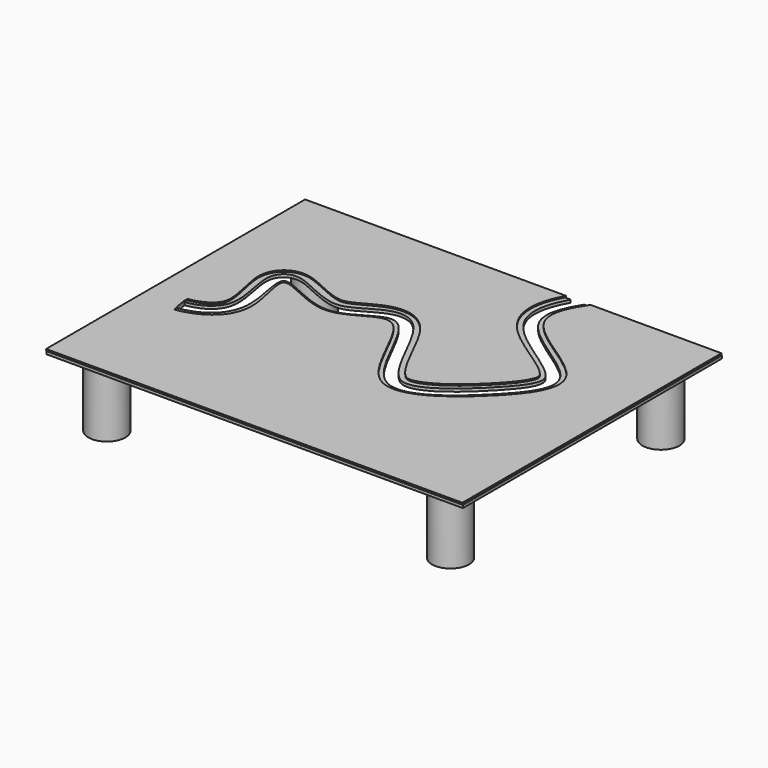
from build123d import *

# Parameters (mm, degrees)
F0_W          = 900
F0_H          = 700
F2_DEPTH      = 3
F3_DEPTH      = 25
F3_DEPTH_BACK = 25
F6_DEPTH      = 25
F6_DEPTH_BACK = 25
F7_W          = 900
F7_H          = 700
F9_DEPTH      = 6
F11_R         = 40
F12_DEPTH     = 150


# Not quite as in the source:
# - the dataset's text gives a spline's control points without its knots; the knots are read off the source's solid


with BuildPart() as f2:
    # F0 (on Top) → F2 (new body)
    with BuildSketch(Plane.XY):
        with Locations((136.779838565, 140.37967287)):
            Rectangle(F0_W, F0_H)
    extrude(amount=F2_DEPTH)

    # F1 (on Top) → F3 (cut, two sides)
    with BuildSketch(Plane.XY) as f3_sk:
        with BuildLine():
            Line((-241.4856788522, 82.2124957097), (-234.3062907457, 37.7888940275))
            add(Edge.make_bspline(
                [(-234.3062907457, 37.7888940275), (-183.2200698821, 46.0450414938), (-107.8197896412, 102.2279372719), (-192.2750551174, 283.579620296), (-24.0171318012, 149.9224145171), (99.4434854713, 307.8000943084), (175.8744786158, -38.137750164), (392.3120352571, 121.8215640239), (495.7588052716, 272.9639793915), (212.09229922, 380.1642280608), (301.8253737576, 491.1332534511), (345.4286754131, 545.0569987297)],
                knots=[0, 0, 0, 0, 0.1005186811, 0.1948714664, 0.2944457767, 0.3919205483, 0.524446972, 0.6500546131, 0.7560619639, 0.8852543369, 1, 1, 1, 1], degree=3))
            Line((345.4286754131, 545.0569987297), (310.4370311075, 573.3516064985))
            add(Edge.make_bspline(
                [(-241.4856788522, 82.2124957097), (-235.5376995244, 83.1737606775), (-227.1834080935, 85.1443072797), (-217.474364878, 88.6042185531), (-210.9663273096, 91.5416769635), (-205.2747075425, 94.7414795634), (-200.4160544418, 98.1187472011), (-196.373293023, 101.5953254918), (-193.0908775239, 105.1164927775), (-190.4790946185, 108.673215132), (-188.772395717, 111.7142206402), (-187.6443639611, 114.2600259837), (-186.91078749, 116.2492961693), (-186.2869465038, 118.3436017222), (-185.8604232074, 120.1988345417), (-185.5789375302, 121.7627021332), (-185.3991590865, 122.9783217928), (-185.252302169, 124.2414938638), (-185.1405994233, 125.5490498855), (-185.059563113, 126.9970714119), (-185.0000994287, 129.0879426638), (-185.0248632154, 131.9899533939), (-185.2286698235, 135.8675595467), (-185.6086882806, 140.0794825573), (-186.1581698074, 144.5682595729), (-187.0987121971, 150.8533570489), (-188.6205679067, 159.1522141918), (-190.8240279465, 169.5043124094), (-192.8083784067, 178.2695336381), (-194.3818406654, 185.3095616522), (-195.5285456157, 190.6070149505), (-196.6143456264, 195.9387036323), (-197.6084875244, 201.3452092887), (-198.4727294543, 206.9018156809), (-199.1496740668, 212.7389962035), (-199.4764712019, 218.0162233827), (-199.4894720296, 222.6632212336), (-199.3258979633, 226.4234804566), (-198.919614654, 230.5290516319), (-198.1659289654, 235.0572516522), (-196.9118918995, 240.0783575162), (-194.9451306123, 245.6253274688), (-192.4879995558, 250.6392221678), (-189.898614037, 254.7703034363), (-187.6218228143, 257.8777610524), (-184.9992992364, 260.934338153), (-182.0377655849, 263.8704376875), (-179.3129029064, 266.1548327791), (-177.000331504, 267.8542399638), (-174.6237907367, 269.4492377395), (-171.6062006951, 271.2068826251), (-167.9761634622, 272.9460428746), (-164.409661789, 274.3311498765), (-159.8065692755, 275.749902793), (-154.4349269126, 276.8203829827), (-148.7149350442, 277.3109893938), (-143.6791934777, 277.2781780434), (-139.2282351443, 276.9098327801), (-135.2505889333, 276.3274056454), (-131.6452560188, 275.6060761092), (-128.327829438, 274.7915830848), (-124.1994201874, 273.6177648935), (-119.454378243, 272.0297965106), (-114.1330202601, 269.9985841874), (-109.0163936944, 267.8708559657), (-104.0042481448, 265.6683344255), (-99.0398525291, 263.4119036969), (-94.0934068391, 261.1245526128), (-87.5071738324, 258.0675515109), (-79.2894636179, 254.301217329), (-69.5603592504, 250.1084557216), (-61.7384184503, 247.0939974118), (-55.7995425295, 245.0842808334), (-51.5499774528, 243.8013204219), (-47.5536122712, 242.7614646682), (-43.8633351999, 241.9756441117), (-41.0890345702, 241.5330763696), (-39.0767461943, 241.2996839349), (-37.6771518248, 241.1816399507), (-36.3922517161, 241.116479596), (-35.4214542607, 241.1018193712), (-34.7043651988, 241.1108325263), (-34.2011207672, 241.1268350515), (-33.6853437819, 241.1532206705), (-32.9848262391, 241.2026104861), (-32.080215541, 241.2918119898), (-30.9425191435, 241.4457711216), (-29.747492374, 241.6498724502), (-28.0732155104, 241.9930222828), (-25.822720168, 242.5627626208), (-21.880330047, 243.7981397699), (-16.331982542, 245.9761062402), (-8.8118359212, 249.5607949136), (-0.5434559099, 253.9526763782), (8.4508129905, 258.9262639267), (16.6403545663, 263.3417972682), (23.7599841554, 266.8841366803), (29.4467345634, 269.4962211057), (35.5566372376, 272.0010306462), (42.1823374373, 274.311405811), (49.4236395705, 276.3023826176), (57.3672041666, 277.795696083), (66.0465099256, 278.5509411968), (75.3837631228, 278.2821676865), (83.5113265637, 276.9778692101), (89.2081655274, 275.4330144664), (92.4367063904, 274.3708027239), (94.8382851466, 273.4852798104), (96.8161375588, 272.6754654295), (98.3841938016, 271.9843530185), (99.9262943401, 271.2721286966), (101.8038878917, 270.3453559302), (104.702705147, 268.7934917732), (108.1317869173, 266.7405344791), (111.9541425106, 264.1395026786), (115.5087239258, 261.4346763787), (119.927069824, 257.7228957042), (124.9169432693, 252.9328275462), (130.2508034542, 247.026543135), (135.0896327978, 240.9927455699), (139.554556696, 234.8416200953), (145.1283850319, 226.4875741975), (151.5589218926, 215.7632245239), (158.7710272688, 202.497891756), (165.6801971146, 188.9538806141), (172.4151365402, 175.2994869993), (179.0582911899, 161.7422451206), (185.660525585, 148.5206349377), (192.2444338178, 135.8994918833), (198.8008182512, 124.1678836236), (205.2768380346, 113.6369815809), (210.5101981, 106.1358052224), (214.4899104198, 101.0609993718), (217.3303617383, 97.7534217065), (219.978464374, 94.9733838681), (222.3765020584, 92.7378899598), (224.1137016073, 91.3274700325), (225.3142899389, 90.4567825785), (226.1163341361, 89.924057213), (226.8029845386, 89.5091405515), (227.4733439715, 89.1430138534), (228.1291176651, 88.822150909), (228.9996846256, 88.4432304879), (230.1054945245, 88.0467609434), (231.54537094, 87.6664964427), (233.1753732843, 87.3794091452), (235.057273097, 87.2021281247), (237.2335796296, 87.1635396823), (240.55731177, 87.3413929062), (245.5227987888, 88.079008451), (252.6791739242, 89.9923664451), (260.8301872351, 93.0264381942), (269.7570797741, 97.1825815618), (279.2556215065, 102.4009159936), (289.1468102787, 108.584934908), (299.2760739512, 115.6176345184), (309.5093899796, 123.3712014191), (319.7287874812, 131.7124258746), (329.8286859902, 140.5058445218), (338.0648038503, 148.0964177817), (344.5013770548, 154.2589683131), (348.4500767297, 158.1321041895), (351.5636214838, 161.2392515861), (354.6286384304, 164.3330415235), (358.3546871655, 168.163507658), (362.6480774345, 172.6981225537), (368.1173165148, 178.6510472941), (374.4439024175, 185.8985119346), (381.1201011492, 194.2088317575), (386.7882817119, 202.0338405705), (391.3723846707, 209.2487053252), (394.8283570488, 215.7004013288), (397.1689795838, 221.2164346332), (398.274140703, 224.8961691748), (398.7586304729, 227.2523477751), (398.9589780282, 228.7346603805), (399.033607176, 229.9543070221), (399.0177225056, 230.952451348), (398.9374713249, 231.7885688151), (398.8035372952, 232.5375385066), (398.6059933192, 233.282855915), (398.3615456687, 233.9702274749), (398.0917291127, 234.596295897), (397.885446547, 235.0253148368), (397.6933380765, 235.3947640399), (397.5351601954, 235.6845823574), (397.3594254936, 235.9919532357), (397.0874783947, 236.4470374628), (396.679784191, 237.0891477727), (395.8733663132, 238.2656919148), (394.567493912, 239.9926785021), (392.5131211223, 242.4074256407), (389.137265676, 246.0021498199), (383.7741089396, 251.0640022626), (375.751488869, 257.7405013236), (366.417496646, 264.8362812315), (356.0404038889, 272.2467658517), (344.8731898776, 279.9209527707), (333.1509121216, 287.8448474083), (321.0910339513, 296.0335168672), (308.893794176, 304.5289467569), (296.7425913103, 313.4033633299), (284.8049272706, 322.7684284522), (273.237915057, 332.7926592747), (264.0409228143, 341.9040126463), (257.0563649981, 349.8326975335), (252.0449681123, 356.1585682546), (248.1020472958, 361.7995109897), (245.1253394442, 366.5665889108), (242.9935925432, 370.2770521418), (241.3129881952, 373.4859400827), (240.0325980452, 376.1290050305), (238.8113517142, 378.7924683854), (237.3946194858, 382.1615894078), (235.3686208631, 387.6220814248), (233.2949562773, 394.552809555), (231.546773022, 402.9453959487), (230.5193972595, 411.3225036077), (230.1719914596, 419.6044271535), (230.4480888242, 427.7291455333), (231.5621988176, 438.2982923287), (234.1862414869, 450.9526422368), (238.8303853448, 465.2427656184), (244.6130062197, 478.7677873011), (251.2809191489, 491.6831883403), (258.6500420567, 504.1296805595), (266.5761934981, 516.2184522105), (274.935846315, 528.0312592745), (283.6149215817, 539.6249662726), (295.464949001, 554.8390039644), (304.4995700078, 566.0088107058), (310.4370311075, 573.3516064985)],
                knots=[0, 0, 0, 0, 0.015625, 0.0234375, 0.03125, 0.0390625, 0.046875, 0.0546875, 0.0625, 0.0703125, 0.078125, 0.08203125, 0.0859375, 0.08984375, 0.09375, 0.095703125, 0.09765625, 0.099609375, 0.1015625, 0.103515625, 0.10546875, 0.109375, 0.11328125, 0.1171875, 0.12109375, 0.125, 0.1328125, 0.140625, 0.1484375, 0.15234375, 0.15625, 0.16015625, 0.1640625, 0.16796875, 0.171875, 0.17578125, 0.177734375, 0.1796875, 0.181640625, 0.18359375, 0.185546875, 0.1875, 0.189453125, 0.1904296875, 0.19140625, 0.1923828125, 0.193359375, 0.1943359375, 0.1948242188, 0.1953125, 0.1962890625, 0.197265625, 0.1982421875, 0.19921875, 0.201171875, 0.203125, 0.205078125, 0.20703125, 0.208984375, 0.2109375, 0.212890625, 0.21484375, 0.21875, 0.22265625, 0.2265625, 0.23046875, 0.234375, 0.23828125, 0.2421875, 0.25, 0.2578125, 0.265625, 0.26953125, 0.2734375, 0.27734375, 0.28125, 0.28515625, 0.287109375, 0.2890625, 0.291015625, 0.29296875, 0.2939453125, 0.294921875, 0.2958984375, 0.296875, 0.298828125, 0.30078125, 0.302734375, 0.3046875, 0.30859375, 0.3125, 0.3203125, 0.328125, 0.3359375, 0.34375, 0.3515625, 0.35546875, 0.359375, 0.36328125, 0.3671875, 0.37109375, 0.375, 0.37890625, 0.3828125, 0.38671875, 0.388671875, 0.3896484375, 0.390625, 0.3916015625, 0.3920898438, 0.392578125, 0.3935546875, 0.39453125, 0.396484375, 0.3984375, 0.400390625, 0.40234375, 0.40625, 0.41015625, 0.4140625, 0.41796875, 0.421875, 0.4296875, 0.4375, 0.4453125, 0.453125, 0.4609375, 0.46875, 0.4765625, 0.484375, 0.4921875, 0.5, 0.50390625, 0.5078125, 0.51171875, 0.515625, 0.51953125, 0.521484375, 0.5234375, 0.525390625, 0.52734375, 0.529296875, 0.53125, 0.53515625, 0.5390625, 0.54296875, 0.546875, 0.55078125, 0.5546875, 0.5625, 0.5703125, 0.578125, 0.5859375, 0.59375, 0.6015625, 0.609375, 0.6171875, 0.625, 0.6328125, 0.640625, 0.64453125, 0.6484375, 0.650390625, 0.65234375, 0.65625, 0.66015625, 0.6640625, 0.671875, 0.6796875, 0.6875, 0.6953125, 0.703125, 0.7109375, 0.71875, 0.72265625, 0.7265625, 0.73046875, 0.734375, 0.73828125, 0.7421875, 0.74609375, 0.75, 0.751953125, 0.75390625, 0.7548828125, 0.755859375, 0.7568359375, 0.7578125, 0.759765625, 0.76171875, 0.765625, 0.76953125, 0.7734375, 0.78125, 0.7890625, 0.796875, 0.8046875, 0.8125, 0.8203125, 0.828125, 0.8359375, 0.84375, 0.8515625, 0.859375, 0.8671875, 0.87109375, 0.875, 0.87890625, 0.880859375, 0.8828125, 0.884765625, 0.8857421875, 0.88671875, 0.888671875, 0.890625, 0.89453125, 0.8984375, 0.90234375, 0.90625, 0.91015625, 0.9140625, 0.921875, 0.9296875, 0.9375, 0.9453125, 0.953125, 0.9609375, 0.96875, 0.9765625, 0.984375, 1, 1, 1, 1], degree=3))
        make_face()
    extrude(amount=F3_DEPTH, mode=Mode.SUBTRACT)
    extrude(f3_sk.sketch, amount=-F3_DEPTH_BACK, mode=Mode.SUBTRACT)


with BuildPart() as f2_1:
    # F5: moved
    add(f2.part.moved(Location((-139, -139, 6))))


with BuildPart() as f6:
    # F4 (on Top) → F6 (new body, two sides)
    with BuildSketch(Plane.XY) as f6_sk:
        with BuildLine():
            Line((-333.2689129169, -208.5999996712), (-329.2803639689, -233.2797783835))
            add(Edge.make_bspline(
                [(-329.2803639689, -233.2797783835), (-279.6440862088, -225.2579591544), (-215.0591975226, -169.0019007955), (-290.3221170229, 10.7279443108), (-115.933229477, -128.5278182105), (8.6171027688, 40.169951089), (91.4360122328, -317.6582258257), (294.4798541771, -146.0859910696), (390.4461045585, -16.0719332642), (105.2391975094, 95.5185231878), (204.8334747082, 217.5691570301), (250.45460219, 273.9883263187)],
                knots=[0, 0, 0, 0, 0.0976657324, 0.1914809372, 0.2938646504, 0.3927571199, 0.5271537272, 0.6507806642, 0.749994953, 0.8799442629, 1, 1, 1, 1], degree=3))
            Line((250.45460219, 273.9883263187), (231.014799798, 289.707552857))
            add(Edge.make_bspline(
                [(-333.2689129169, -208.5999996712), (-326.5356582324, -207.5118247648), (-317.1931037284, -205.2387950425), (-306.3838909726, -201.131018164), (-299.1159354338, -197.5685255044), (-292.6875905846, -193.5780513816), (-287.0795024379, -189.2040888935), (-282.2539728874, -184.4715031927), (-278.1616343726, -179.3755889151), (-274.7548284297, -173.8762725729), (-272.004457018, -167.9012394607), (-270.2621207217, -162.4489840488), (-269.3492323658, -158.3439603506), (-268.9196013639, -155.9107657182), (-268.6445813298, -154.0412952716), (-268.4179617417, -152.1250200421), (-268.2708607574, -150.4920692989), (-268.178315106, -149.1553098982), (-268.1017791313, -147.787649081), (-268.0366959253, -146.0273373624), (-268.0074636443, -143.83809812), (-268.0330013502, -140.8251744651), (-268.1836815232, -136.8974040515), (-268.5425410407, -131.9712532313), (-269.2358295256, -125.1762280136), (-270.4560911543, -116.3586946136), (-272.3017603747, -105.545902828), (-274.3259989971, -94.7403069697), (-276.3185069389, -84.1277531076), (-277.772685312, -75.5387465003), (-278.6910565664, -68.799797955), (-279.2187644678, -63.7788161512), (-279.5350356557, -58.733830778), (-279.5604611746, -53.5647284485), (-279.2250415257, -49.0206940891), (-278.6023825049, -45.1323212194), (-277.8982640923, -42.0603377083), (-276.8797273076, -38.8121645014), (-275.4455548583, -35.3892511345), (-273.4790588951, -31.8374466759), (-271.305823316, -28.8665182353), (-269.2236062579, -26.5816714906), (-267.4957329052, -24.9446019313), (-265.9272233847, -23.6693040063), (-264.6061679224, -22.7168534474), (-263.5845965554, -22.0387788556), (-262.5400095899, -21.4024713172), (-261.1379217102, -20.6202936087), (-259.3723656238, -19.7624478141), (-257.2664768815, -18.9191927957), (-254.5077179753, -18.0245960695), (-251.2000220802, -17.2947134288), (-247.526764406, -16.8905642308), (-244.1461911465, -16.8266916994), (-241.0218040198, -17.0055225982), (-238.1058387703, -17.3595544011), (-234.4344132952, -18.0062082748), (-230.1461571265, -19.0650837496), (-225.2401991321, -20.6081155776), (-220.428560194, -22.3650098202), (-215.6241958309, -24.2977102764), (-209.1635726945, -27.0686912343), (-200.91533098, -30.8248650185), (-190.6992823023, -35.5633740418), (-180.2474658182, -40.2795972838), (-169.7035594185, -44.7101422758), (-159.2590572075, -48.5915934212), (-150.833086294, -51.1595912285), (-144.3969270885, -52.708623803), (-139.7597894843, -53.5984287402), (-135.350217645, -54.2021923049), (-131.8947581809, -54.4618466023), (-129.2773886965, -54.5250055118), (-127.3886195937, -54.5012672263), (-125.5834761423, -54.4084821332), (-123.75735039, -54.2430127225), (-121.9179256246, -54.0060449492), (-119.4386939412, -53.5950915733), (-115.0236778915, -52.6281983161), (-108.464450337, -50.5461688208), (-100.209458435, -47.0145503997), (-91.6473177788, -42.6292695447), (-82.8356633205, -37.6323659906), (-73.7820326342, -32.2980788941), (-64.4204788343, -26.9162564968), (-56.2244895109, -22.6463808947), (-49.2756699808, -19.5487355759), (-43.8133941483, -17.4497347779), (-38.0428319595, -15.6577145741), (-31.9100593387, -14.2848925391), (-25.3863705909, -13.4787706401), (-18.5000233839, -13.4165023579), (-12.557265223, -14.133129136), (-7.7865894592, -15.2265427799), (-4.8246097736, -16.1301935238), (-2.4830188095, -16.984188282), (-0.7427660824, -17.6899007664), (0.9709845891, -18.4568454065), (3.1885919534, -19.5421936723), (5.8485426274, -21.0115303516), (9.8718071452, -23.5627825113), (14.5000714326, -27.0687833334), (19.5365876981, -31.6576976572), (24.1739882822, -36.5623991895), (28.5076750141, -41.7464765079), (32.6112471084, -47.1880102691), (37.8488651353, -54.764030926), (44.0654277581, -64.7959256173), (51.2201351181, -77.5865758044), (58.2026287306, -90.9485676633), (65.1030299231, -104.6722368616), (71.9847087497, -118.5258924104), (78.8933104853, -132.2605289934), (85.8592210003, -145.6123778219), (92.8961025164, -158.3039513189), (99.9953000632, -170.0442708674), (107.1143439792, -180.530730928), (112.9853173881, -187.9673444171), (117.5571297552, -192.9928132518), (120.891347435, -196.2718180315), (123.5607943849, -198.5789440356), (125.6110125922, -200.1666005585), (127.1013954479, -201.2296275031), (128.299871881, -202.0106634877), (129.2319913269, -202.5751821399), (130.1420372188, -203.0981419586), (131.2710187578, -203.6944665479), (132.626458923, -204.3302155974), (133.9864461835, -204.8908623689), (135.8156146818, -205.545292611), (138.1487884217, -206.198760127), (141.077635188, -206.7370218737), (145.2141858408, -207.1274073481), (150.9064499461, -206.9767427556), (158.6590034827, -205.6449354418), (167.244272616, -203.074417377), (176.5043495372, -199.2617251909), (186.269555269, -194.2698704354), (196.3839518787, -188.2045424102), (206.7110295818, -181.1952498955), (217.1322533607, -173.3837647463), (227.5435683457, -164.9175624249), (237.8519285523, -155.9463690586), (247.9727234425, -146.6201938313), (256.1846315059, -138.6774946859), (262.5848873219, -132.2944036856), (267.2896553578, -127.5126499147), (271.8985046876, -122.748219897), (276.3517380743, -118.064097177), (280.6360934064, -113.4597602), (286.1050318739, -107.4319261502), (292.4503775362, -100.1139582853), (299.1710967524, -91.7191679074), (304.8952626236, -83.7698370339), (309.5342332929, -76.3475286822), (313.0297660901, -69.5576730595), (315.3796022741, -63.5166343333), (316.4534174009, -59.1803878595), (316.8684624481, -56.1104390775), (316.9825551901, -53.9805609293), (316.9189582881, -51.9841685855), (316.6870514368, -50.0672519618), (316.2805485965, -48.1671369792), (315.7761402691, -46.5443817923), (315.2528137353, -45.1946320684), (314.7940046118, -44.150856615), (314.3510194684, -43.2510672458), (313.9563962067, -42.5107950014), (313.6403277182, -41.946580014), (313.2996180656, -41.3666861232), (312.8071634118, -40.5653642298), (312.1212354569, -39.5166101946), (311.1830626083, -38.1877669006), (309.7784964594, -36.3308443648), (307.7357978991, -33.8650208604), (304.8404403301, -30.7178973681), (301.5251654901, -27.4183194333), (296.5833748239, -22.8530326503), (289.5064042219, -16.8926708352), (279.8319575373, -9.4512466565), (269.227680549, -1.7805411734), (257.934312506, 6.0926856509), (246.1812875466, 14.1644513549), (234.1876053412, 22.4474173419), (222.1627658357, 30.9689201568), (210.3075244762, 39.7718879334), (198.8148664416, 48.9186823586), (187.8729843469, 58.4986195172), (179.3718553715, 66.9485512729), (173.0482225424, 74.0787256506), (168.5766093857, 79.6400266203), (164.4138513635, 85.4456908838), (161.2410767319, 90.514082676), (158.9095794021, 94.7226214256), (157.2734640868, 97.9573725172), (155.75735069, 101.2794930253), (154.3903989976, 104.6366271066), (153.1706645122, 108.0265936891), (151.7416942377, 112.581548034), (149.756114357, 120.6251220695), (148.3634532991, 132.2007283871), (148.7712889539, 145.9093868829), (150.9390302606, 159.2673485535), (154.5610013717, 172.2378616731), (159.3830697519, 184.856918191), (165.2034437031, 197.1847219475), (171.8581554162, 209.2797407613), (181.656654805, 225.1567879701), (195.3201464248, 244.6214659901), (213.0280067843, 267.48337337), (225.0836440416, 282.3725548162), (231.014799798, 289.707552857)],
                knots=[0, 0, 0, 0, 0.015625, 0.0234375, 0.03125, 0.0390625, 0.046875, 0.0546875, 0.0625, 0.0703125, 0.078125, 0.0859375, 0.08984375, 0.091796875, 0.09375, 0.095703125, 0.09765625, 0.0986328125, 0.099609375, 0.1015625, 0.103515625, 0.10546875, 0.109375, 0.11328125, 0.1171875, 0.125, 0.1328125, 0.140625, 0.1484375, 0.15625, 0.16015625, 0.1640625, 0.16796875, 0.171875, 0.17578125, 0.177734375, 0.1796875, 0.181640625, 0.18359375, 0.185546875, 0.1875, 0.1884765625, 0.189453125, 0.1904296875, 0.1909179688, 0.19140625, 0.1918945312, 0.1923828125, 0.193359375, 0.1943359375, 0.1953125, 0.197265625, 0.19921875, 0.201171875, 0.203125, 0.205078125, 0.20703125, 0.2109375, 0.21484375, 0.21875, 0.22265625, 0.2265625, 0.234375, 0.2421875, 0.25, 0.2578125, 0.265625, 0.2734375, 0.27734375, 0.28125, 0.28515625, 0.2890625, 0.291015625, 0.29296875, 0.294921875, 0.296875, 0.298828125, 0.30078125, 0.3046875, 0.3125, 0.3203125, 0.328125, 0.3359375, 0.34375, 0.3515625, 0.359375, 0.36328125, 0.3671875, 0.37109375, 0.375, 0.37890625, 0.3828125, 0.38671875, 0.388671875, 0.390625, 0.3916015625, 0.392578125, 0.3935546875, 0.39453125, 0.396484375, 0.3984375, 0.40234375, 0.40625, 0.41015625, 0.4140625, 0.41796875, 0.421875, 0.4296875, 0.4375, 0.4453125, 0.453125, 0.4609375, 0.46875, 0.4765625, 0.484375, 0.4921875, 0.5, 0.5078125, 0.51171875, 0.515625, 0.51953125, 0.521484375, 0.5234375, 0.525390625, 0.5263671875, 0.52734375, 0.529296875, 0.53125, 0.533203125, 0.53515625, 0.5390625, 0.54296875, 0.546875, 0.5546875, 0.5625, 0.5703125, 0.578125, 0.5859375, 0.59375, 0.6015625, 0.609375, 0.6171875, 0.625, 0.6328125, 0.640625, 0.64453125, 0.6484375, 0.65234375, 0.65625, 0.66015625, 0.6640625, 0.671875, 0.6796875, 0.6875, 0.6953125, 0.703125, 0.7109375, 0.71875, 0.72265625, 0.7265625, 0.73046875, 0.734375, 0.73828125, 0.7421875, 0.744140625, 0.74609375, 0.748046875, 0.7490234375, 0.75, 0.7509765625, 0.751953125, 0.75390625, 0.755859375, 0.7578125, 0.76171875, 0.765625, 0.76953125, 0.7734375, 0.78125, 0.7890625, 0.796875, 0.8046875, 0.8125, 0.8203125, 0.828125, 0.8359375, 0.84375, 0.8515625, 0.859375, 0.86328125, 0.8671875, 0.87109375, 0.875, 0.876953125, 0.87890625, 0.880859375, 0.8828125, 0.884765625, 0.88671875, 0.890625, 0.8984375, 0.90625, 0.9140625, 0.921875, 0.9296875, 0.9375, 0.9453125, 0.953125, 0.96875, 0.984375, 1, 1, 1, 1], degree=3))
        make_face()
    extrude(amount=F6_DEPTH)
    extrude(f6_sk.sketch, amount=-F6_DEPTH_BACK)


with BuildPart() as f6_1:
    # F8: moved
    add(f6.part.moved(Location((-47, 144, 0))))


with BuildPart() as f9:
    # F7 (on Top) → F9 (new body)
    with BuildSketch(Plane.XY):
        Rectangle(F7_W, F7_H)
    extrude(amount=F9_DEPTH)

    # F10: cut F6
    add(f6_1.part, mode=Mode.SUBTRACT)


with BuildPart() as f2_2:
    add(f2_1.part)

    # F10: cut F6
    add(f6_1.part, mode=Mode.SUBTRACT)


with BuildPart() as f12:
    # F11 (on face) → F12 (new body)
    with BuildSketch(Plane(origin=(0, 0, 0), x_dir=(1, 0, 0), z_dir=(0, 0, -1))):
        with Locations((-634.1957449913, 220.3838676214)):
            Circle(F11_R)
    extrude(amount=F12_DEPTH)


with BuildPart() as f12_1:
    # F13: moved
    add(f12.part.moved(Location((258, -59, 0))))


with BuildPart() as f14_1:
    # F14: copy of F12
    add(f12_1.part.moved(Location((0, 561, 0))))


with BuildPart() as f15_1:
    # F15: copy of F12
    add(f12_1.part.moved(Location((743, 0, 0))))


with BuildPart() as f16_1:
    # F16: copy of F14_1
    add(f14_1.part.moved(Location((749, 0, 0))))


solid = Compound([f9.part, f2_2.part, f12_1.part, f14_1.part, f15_1.part, f16_1.part])
